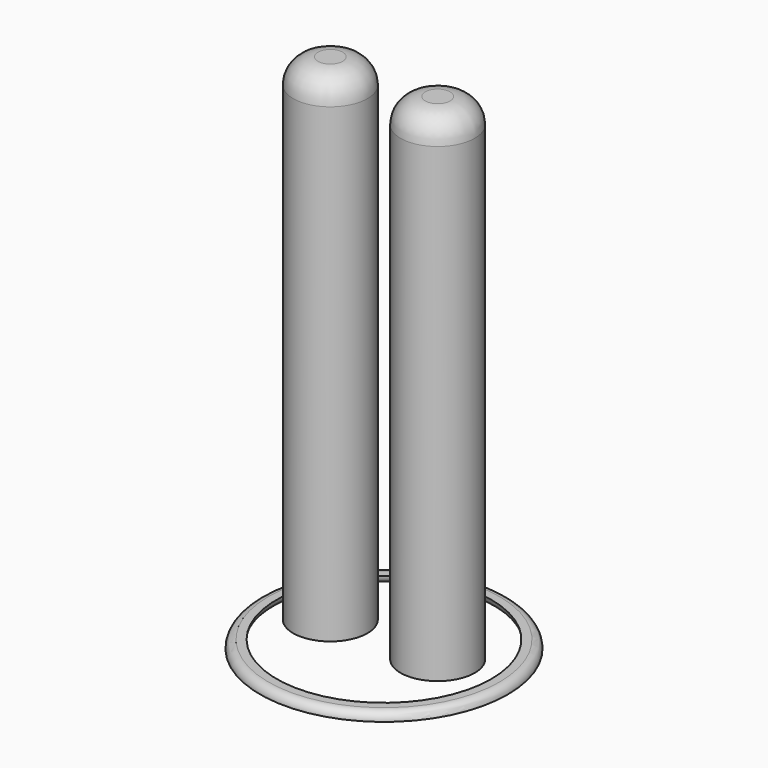
from build123d import *

# Parameters (mm, degrees)
F0_R     = 75
F0_R_2   = 65
F1_DEPTH = 5
F2_R     = 4.99999
F4_DEPTH = 300


# Not quite as in the source:
# - a fillet or chamfer that OpenCascade refuses, or shapes differently, is made with other operations: its cross-section is extruded or revolved along the edge and cut away or added
# - a fillet or chamfer is up to 0.001 mm smaller than in the source, because OpenCascade refuses the exact size


with BuildPart() as f1:
    # F0 (on Top) → F1 (new body)
    with BuildSketch(Plane.XY):
        Circle(F0_R)
        Circle(F0_R_2, mode=Mode.SUBTRACT)
    extrude(amount=F1_DEPTH)

    # F2 (radius 5 in the source; OpenCascade refuses exactly that, so slightly less here)
    f2_edges = [f1.edges().sort_by_distance(p)[0] for p in [
        (-75, 0, 5),
        (-65, 0, 0),
    ]]
    fillet(f2_edges, radius=F2_R)


with BuildPart() as f4:
    # F3 (on face) → F4 (new body)
    with BuildSketch(Plane.XY.offset(5)):
        with BuildLine():
            ThreePointArc((-10, 0), (-32.5, 22.5), (-55, 0))
            ThreePointArc((-55, 0), (-32.5, -22.5), (-10, 0))
        make_face()
    extrude(amount=F4_DEPTH)

    # F5: fillet of radius 15 on 1 edges, made by hand

    # F5_s1 → F5_t2 (revolve, cut)
    with BuildSketch(Plane.XZ):
        with BuildLine():
            ThreePointArc((-10, 290), (-14.3933982822, 300.6066017178), (-25, 305))
            Line((-25, 305), (-10, 305))
            Line((-10, 305), (-10, 290))
        make_face()
    revolve(axis=Axis((-32.5, 0, 305), (0, 0, -1)), mode=Mode.SUBTRACT)


with BuildPart() as f4b:
    # F3 (on face) → F4, piece 2 (new body)
    with BuildSketch(Plane.XY.offset(5)):
        with BuildLine():
            ThreePointArc((10, 0), (32.5, -22.5), (55, 0))
            ThreePointArc((55, 0), (32.5, 22.5), (10, 0))
        make_face()
    extrude(amount=F4_DEPTH)

    # F5#2: fillet of radius 15 on 1 edges, made by hand

    # F5_2_s1 → F5_2_t2 (revolve, cut)
    with BuildSketch(Plane.XZ):
        with BuildLine():
            ThreePointArc((55, 290), (50.6066017178, 300.6066017178), (40, 305))
            Line((40, 305), (55, 305))
            Line((55, 305), (55, 290))
        make_face()
    revolve(axis=Axis((32.5, 0, 305), (0, 0, -1)), mode=Mode.SUBTRACT)


solid = Compound([f1.part, f4.part, f4b.part])
